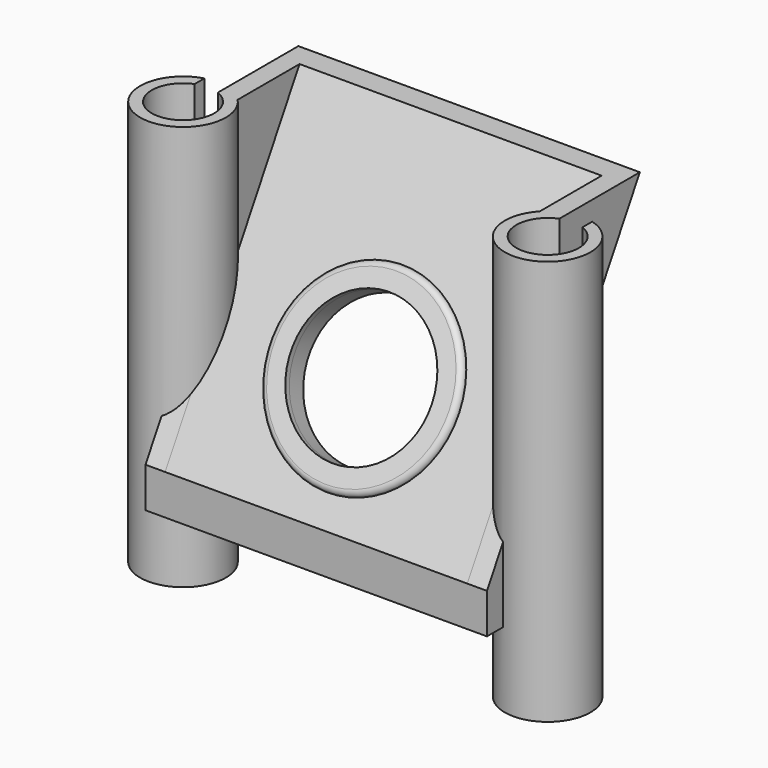
from build123d import *

# Parameters (mm, degrees)
F0_R      = 3.7
F0_R_2    = 2.7
F1_DEPTH  = 35
F2_W      = 2
F2_H      = 6.1218521535
F3_DEPTH  = 35.001
F6_W      = 26.1
F6_H      = 2
F8_W      = 26.1
F8_H      = 2
F11_DEPTH = 1.7
F13_DEPTH = 1.7
F14_R     = 6.1
F15_DEPTH = 19.2330509442
F14_R_2   = 8.1
F16_DEPTH = 0.5
F17_R     = 0.49999
F19_DEPTH = 26.1
F21_DEPTH = 1.7
F23_DEPTH = 1.7


# Not quite as in the source:
# - a fillet or chamfer is up to 0.001 mm smaller than in the source, because OpenCascade refuses the exact size


with BuildPart() as f1:
    # F0 (on Top) → F1 (new body)
    with BuildSketch(Plane.XY):
        with Locations((-15.75, 0)):
            Circle(F0_R)
        with Locations((-15.75, 0)):
            Circle(F0_R_2, mode=Mode.SUBTRACT)
    extrude(amount=F1_DEPTH)

    # F2 (on Top) → F3 (cut, through all)
    with BuildSketch(Plane.XY):
        with Locations((-15.75, 2.7)):
            Rectangle(F2_W, F2_H)
    extrude(amount=F3_DEPTH, mode=Mode.SUBTRACT)


with BuildPart() as f5_1:
    # F5: instance of F1
    add(f1.part.mirror(Plane.YZ))


with BuildPart() as f1_1:
    add(f1.part)

    add(f5_1.part)  # F9 merges F5_1
    # F6 (on Top) → F9 section 0
    with BuildSketch(Plane.XY):
        with Locations((0, -10)):
            Rectangle(F6_W, F6_H)
    # F8 (on offset) → F9 section 1
    with BuildSketch(Plane.XY.offset(35)):
        with Locations((0, 10.2072594216)):
            Rectangle(F8_W, F8_H)
    loft()

    # F10 (on face) → F11 (join, through all)
    with BuildSketch(Plane.YZ.offset(13.05)):
        Polygon((2.5079872408, 19.9324185939), (2.5298221281, 19.9702377282), (11.2072594216, 35), (2.5079872408, 35), align=None)
    extrude(amount=F11_DEPTH)

    # F12 (on face) → F13 (join, through all)
    with BuildSketch(Plane(origin=(-13.05, 0, 0), x_dir=(0, -1, 0), z_dir=(-1, 0, 0))):
        Polygon((-11.2072594216, 35), (-2.5298221281, 19.9702377282), (-2.5079872408, 19.9324185939), (-2.5079872408, 35), align=None)
    extrude(amount=F13_DEPTH)

    # F14 (on face) → F15 (cut, through all)
    with BuildSketch(Plane(origin=(0, -8.25, 4.7631397208), x_dir=(1, 0, 0), z_dir=(0, -0.8660254038, 0.5))):
        with Locations((0, 16.5)):
            Circle(F14_R)
    extrude(amount=-F15_DEPTH, mode=Mode.SUBTRACT)

    # F14 (on face) → F16 (join)
    with BuildSketch(Plane(origin=(0, -8.25, 4.7631397208), x_dir=(1, 0, 0), z_dir=(0, -0.8660254038, 0.5))):
        with Locations((0, 16.5)):
            Circle(F14_R_2)
        with Locations((0, 16.5)):
            Circle(F14_R, mode=Mode.SUBTRACT)
    extrude(amount=F16_DEPTH)

    # F17 (radius 0.5 in the source; OpenCascade refuses exactly that, so slightly less here)
    f17_edges = [f1_1.edges().sort_by_distance(p)[0] for p in [
        (-8.1, -0.433013, 19.302559),
    ]]
    fillet(f17_edges, radius=F17_R)

    # F18 (on face) → F19 (cut, through all)
    with BuildSketch(Plane.YZ.offset(13.05)):
        Polygon((-5.3, 9.8726896031), (-11, 0), (-9, 0), (-5.3, 6.408587988), align=None)
    extrude(amount=-F19_DEPTH, mode=Mode.SUBTRACT)

    # F20 (on face) → F21 (join, through all)
    with BuildSketch(Plane.YZ.offset(13.05)):
        Polygon((-2.5298221281, 14.6707784232), (-5.3, 9.8726896031), (-5.3, 6.408587988), (-2.5298221281, 6.408587988), align=None)
    extrude(amount=F21_DEPTH)

    # F22 (on face) → F23 (join, through all)
    with BuildSketch(Plane(origin=(-13.05, 0, 0), x_dir=(0, -1, 0), z_dir=(-1, 0, 0))):
        Polygon((5.3, 6.408587988), (5.3, 9.8726896031), (2.5298221281, 14.6707784232), (2.5298221281, 6.408587988), align=None)
    extrude(amount=F23_DEPTH)


solid = f1_1.part
